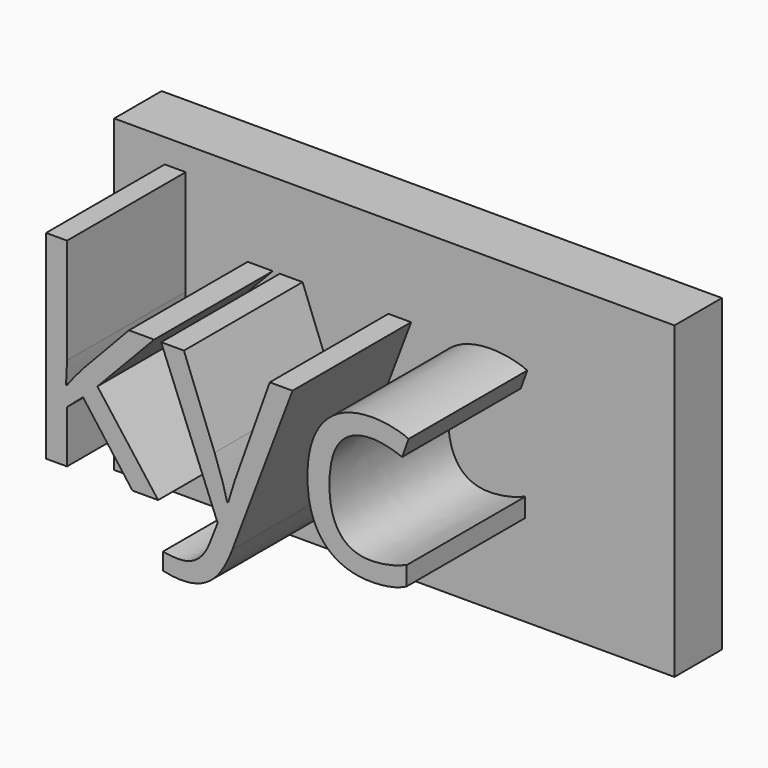
from build123d import *

# Parameters (mm, degrees)
F0_W         = 95.9566906095
F0_H         = 53.0020147562
F1_DEPTH     = 10.16
F2_TEXT_SIZE = 44.8084656253
F3_DEPTH     = 25.4


# Not quite as in the source:
# - Text() gives the source's letters only with a copy of the font that has no kerning and outlines rounded to 1/6400 em; it was checked with that copy


with BuildPart() as f1:
    # F0 (on Front) → F1 (new body)
    with BuildSketch(Plane.XZ):
        with Locations((47.9783453047, 26.5010073781)):
            Rectangle(F0_W, F0_H)
    extrude(amount=F1_DEPTH)

    # F2 (on face) → F3 (join)
    with BuildSketch(Plane.XZ.offset(10.16)):
        with Locations((4.8085870221, 14.8405646905)):
            Text('kyc', F2_TEXT_SIZE, font='Open Sans', text_align=(TextAlign.LEFT, TextAlign.BOTTOM))
    extrude(amount=F3_DEPTH)


solid = f1.part
